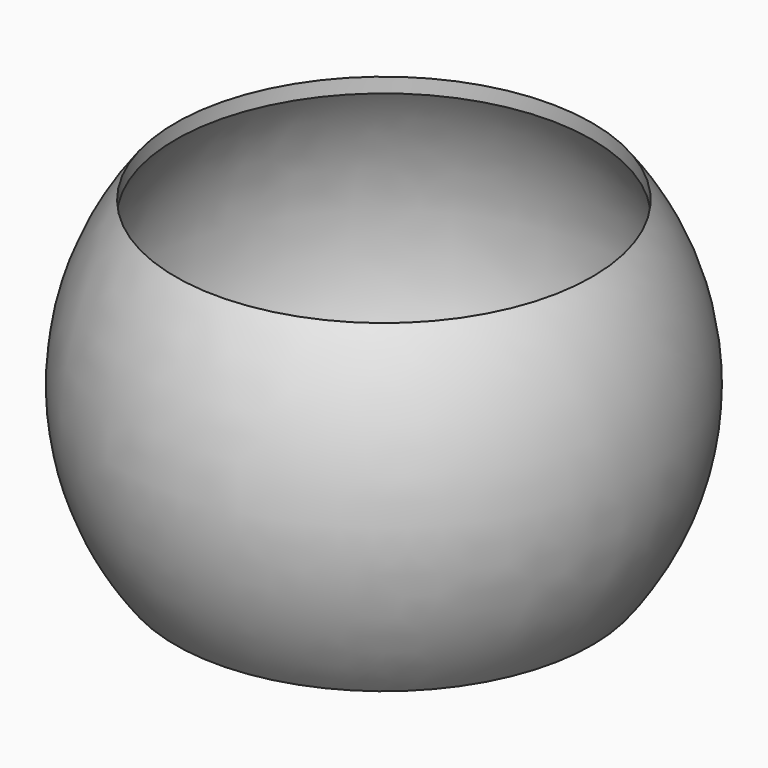
from build123d import *

# Parameters (mm, degrees)
F0_W     = 100
F0_H     = 100
F1_DEPTH = 5
F8_R     = 70.7106781187
F9_DEPTH = 5


with BuildPart() as f1:
    # F0 (on Top) → F1 (new body)
    with BuildSketch(Plane.XY):
        Rectangle(F0_W, F0_H)
    extrude(amount=F1_DEPTH)



with BuildPart() as f7:
    # F4 (on offset) → F7 (revolve)
    with BuildSketch(Plane(origin=(-50, 0, 0), x_dir=(0, -1, 0), z_dir=(-1, 0, 0))):
        with BuildLine():
            Line((50, 5), (50, 0))
            ThreePointArc((50, 0), (74.3303424836, 55.000000824), (49.9999962747, 110))
            Line((49.9999962747, 110), (49.999996444, 105.0000001693))
            ThreePointArc((49.999996444, 105.0000001693), (70.7106769213, 55.0000008211), (50, 5))
        make_face()
    revolve(axis=Axis((0, 0, 56.244302541), (0, 0, 1)))


with BuildPart() as f1_1:
    add(f1.part)

    add(f7.part)  # F9 merges F7
    # F8 (on Top) → F9 (join)
    with BuildSketch(Plane.XY):
        Circle(F8_R)
    extrude(amount=F9_DEPTH)


solid = f1_1.part
